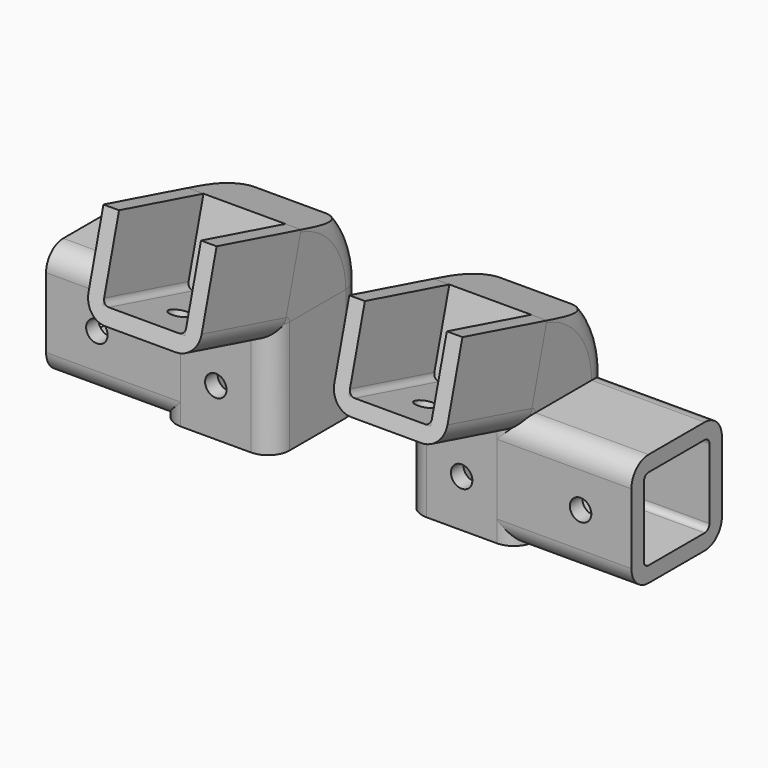
from build123d import *

# Parameters (mm, degrees)
F1_DEPTH  = 29
F3_DEPTH  = 21
F5_DEPTH  = 28
F7_DEPTH  = 28
F9_ANGLE  = 75
F11_DEPTH = 43.3
F12_R     = 2.75
F13_DEPTH = 5
F14_R     = 2.5
F15_DEPTH = 5
F16_W     = 18
F16_H     = 4
F17_DEPTH = 5.5
F18_W     = 1.5
F18_H     = 18
F19_DEPTH = 29
F21_DEPTH = 23.5
F22_R     = 2.75
F23_DEPTH = 15.2


with BuildPart() as f1:
    # F0 (on Top) → F1 (new body)
    with BuildSketch(Plane.XY):
        with BuildLine():
            Line((1.5, -4), (19.5, -4))
            ThreePointArc((19.5, -4), (23.3890872965, -2.3890872965), (25, 1.5))
            Line((25, 1.5), (25, 19.5))
            ThreePointArc((25, 19.5), (23.3890872965, 23.3890872965), (19.5, 25))
            Line((19.5, 25), (1.5, 25))
            ThreePointArc((1.5, 25), (-2.3890872965, 23.3890872965), (-4, 19.5))
            Line((-4, 19.5), (-4, 1.5))
            ThreePointArc((-4, 1.5), (-2.3890872965, -2.3890872965), (1.5, -4))
        make_face()
        with BuildLine():
            Line((19.5, 0), (1.5, 0))
            ThreePointArc((1.5, 0), (0.4393398282, 0.4393398282), (0, 1.5))
            Line((0, 1.5), (0, 19.5))
            ThreePointArc((0, 19.5), (0.4393398282, 20.5606601718), (1.5, 21))
            Line((1.5, 21), (19.5, 21))
            ThreePointArc((19.5, 21), (20.5606601718, 20.5606601718), (21, 19.5))
            Line((21, 19.5), (21, 1.5))
            ThreePointArc((21, 1.5), (20.5606601718, 0.4393398282), (19.5, 0))
        make_face(mode=Mode.SUBTRACT)
    extrude(amount=-F1_DEPTH)

    # F12 (on face) → F13 (cut)
    with BuildSketch(Plane.XZ.offset(4)):
        with Locations((10.5, -16.8672984689)):
            Circle(F12_R)
    extrude(amount=-F13_DEPTH, mode=Mode.SUBTRACT)


with BuildPart() as f3:
    # F2 (on Right) → F3 (new body)
    with BuildSketch(Plane.YZ):
        Polygon((-27.0459231361, 7.2469332629), (0, 0), (5.1763809021, 19.3185165258), (-21.869542234, 26.5654497887), align=None)
    extrude(amount=F3_DEPTH)

    # F6 (on face) → F7 (cut)
    with BuildSketch(Plane(origin=(0, -27.0459231361, 7.2469332629), x_dir=(1, 0, 0), z_dir=(0, -0.9659258263, 0.2588190451))):
        with BuildLine():
            Line((21, 20), (0, 20))
            Line((0, 20), (0, 1.5))
            ThreePointArc((0, 1.5), (0.4393398282, 0.4393398282), (1.5, 0))
            Line((1.5, 0), (19.5, 0))
            ThreePointArc((19.5, 0), (20.5606601718, 0.4393398282), (21, 1.5))
            Line((21, 1.5), (21, 20))
        make_face()
    extrude(amount=-F7_DEPTH, mode=Mode.SUBTRACT)


with BuildPart() as f5:
    # F4 (on face) → F5 (new body)
    with BuildSketch(Plane(origin=(0, -27.0459231361, 7.2469332629), x_dir=(1, 0, 0), z_dir=(0, -0.9659258263, 0.2588190451))):
        with BuildLine():
            Line((0, 1.5), (0, 20))
            Line((0, 20), (-4, 20))
            Line((-4, 20), (-4, 1.5))
            ThreePointArc((-4, 1.5), (-2.3890872965, -2.3890872965), (1.5, -4))
            Line((1.5, -4), (19.5, -4))
            ThreePointArc((19.5, -4), (23.3890872965, -2.3890872965), (25, 1.5))
            Line((25, 1.5), (25, 20))
            Line((25, 20), (21, 20))
            Line((21, 20), (21, 1.5))
            Line((21, 1.5), (21, 0))
            Line((21, 0), (19.5, 0))
            Line((19.5, 0), (1.5, 0))
            Line((1.5, 0), (0, 0))
            Line((0, 0), (0, 1.5))
        make_face()
    extrude(amount=-F5_DEPTH)

    # F14 (on face) → F15 (cut)
    with BuildSketch(Plane(origin=(0, -1.0352761804, -3.8637033052), x_dir=(1, 0, 0), z_dir=(0, -0.2588190451, -0.9659258263))):
        with Locations((10.5, 16.148366034)):
            Circle(F14_R)
    extrude(amount=-F15_DEPTH, mode=Mode.SUBTRACT)


with BuildPart() as f9:
    # F8 (on face) → F9 (revolve)
    with BuildSketch(Plane.XY):
        with BuildLine():
            ThreePointArc((0, 19.5), (0.4393398282, 20.5606601718), (1.5, 21))
            Line((1.5, 21), (19.5, 21))
            ThreePointArc((19.5, 21), (20.5606601718, 20.5606601718), (21, 19.5))
            Line((21, 19.5), (21, 1.5))
            ThreePointArc((21, 1.5), (20.5606601718, 0.4393398282), (19.5, 0))
            Line((19.5, 0), (24.7915026221, 0))
            ThreePointArc((24.7915026221, 0), (24.9476262914, 0.7427894684), (25, 1.5))
            Line((25, 1.5), (25, 19.5))
            ThreePointArc((25, 19.5), (23.3890872965, 23.3890872965), (19.5, 25))
            Line((19.5, 25), (1.5, 25))
            ThreePointArc((1.5, 25), (-2.3890872965, 23.3890872965), (-4, 19.5))
            Line((-4, 19.5), (-4, 1.5))
            ThreePointArc((-4, 1.5), (-3.9476262914, 0.7427894684), (-3.7915026221, 0))
            Line((-3.7915026221, 0), (1.5, 0))
            ThreePointArc((1.5, 0), (0.4393398282, 0.4393398282), (0, 1.5))
            Line((0, 1.5), (0, 19.5))
        make_face()
        with BuildLine():
            Line((19.5, 21), (1.5, 21))
            ThreePointArc((1.5, 21), (0.4393398282, 20.5606601718), (0, 19.5))
            Line((0, 19.5), (0, 1.5))
            ThreePointArc((0, 1.5), (0.4393398282, 0.4393398282), (1.5, 0))
            Line((1.5, 0), (19.5, 0))
            ThreePointArc((19.5, 0), (20.5606601718, 0.4393398282), (21, 1.5))
            Line((21, 1.5), (21, 19.5))
            ThreePointArc((21, 19.5), (20.5606601718, 20.5606601718), (19.5, 21))
        make_face()
    revolve(axis=Axis((10.5, 0, 0), (1, 0, 0)), revolution_arc=F9_ANGLE)

    # F10 (on face) → F11 (cut)
    with BuildSketch(Plane(origin=(-4, 0, 0), x_dir=(0, -1, 0), z_dir=(-1, 0, 0))):
        Polygon((-21.5909180111, 14.9202545633), (-5.1763809021, 19.3185165258), (-5.1763809021, 24.5526935905), (-23.506142199, 23.2962071896), align=None)
    extrude(amount=-F11_DEPTH, mode=Mode.SUBTRACT)


with BuildPart() as f17:
    # F16 (on face) → F17 (new body, symmetric)
    with BuildSketch(Plane.YZ.offset(25)):
        with Locations((10.5, -2)):
            Rectangle(F16_W, F16_H)
        with Locations((10.5, -27)):
            Rectangle(F16_W, F16_H)
        with BuildLine():
            ThreePointArc((-4, -23.5), (-2.3890872965, -27.3890872965), (1.5, -29))
            Line((1.5, -29), (1.5, -25))
            ThreePointArc((1.5, -25), (0.4393398282, -24.5606601718), (0, -23.5))
            Line((0, -23.5), (0, -5.5))
            ThreePointArc((0, -5.5), (0.4393398282, -4.4393398282), (1.5, -4))
            Line((1.5, -4), (1.5, 0))
            ThreePointArc((1.5, 0), (-2.3890872965, -1.6109127035), (-4, -5.5))
            Line((-4, -5.5), (-4, -23.5))
        make_face()
        with BuildLine():
            Line((19.5, -25), (19.5, -29))
            ThreePointArc((19.5, -29), (23.3890872965, -27.3890872965), (25, -23.5))
            Line((25, -23.5), (25, -5.5))
            ThreePointArc((25, -5.5), (23.3890872965, -1.6109127035), (19.5, 0))
            Line((19.5, 0), (19.5, -4))
            ThreePointArc((19.5, -4), (20.5606601718, -4.4393398282), (21, -5.5))
            Line((21, -5.5), (21, -23.5))
            ThreePointArc((21, -23.5), (20.5606601718, -24.5606601718), (19.5, -25))
        make_face()
    extrude(amount=F17_DEPTH, both=True)

    # F18 (on face) → F19 (cut)
    with BuildSketch(Plane(origin=(0, 0, -29), x_dir=(1, 0, 0), z_dir=(0, 0, -1))):
        with BuildLine():
            ThreePointArc((21, -1.5), (20.5606601718, -0.4393398282), (19.5, 0))
            Line((19.5, 0), (19.5, -1.5))
            Line((19.5, -1.5), (21, -1.5))
        make_face()
        with Locations((20.25, -10.5)):
            Rectangle(F18_W, F18_H)
        with BuildLine():
            Line((21, -19.5), (19.5, -19.5))
            Line((19.5, -19.5), (19.5, -21))
            ThreePointArc((19.5, -21), (20.5606601718, -20.5606601718), (21, -19.5))
        make_face()
    extrude(amount=-F19_DEPTH, mode=Mode.SUBTRACT)

    # F20 (on face) → F21 (join)
    with BuildSketch(Plane.YZ.offset(30.5)):
        with BuildLine():
            Line((25, -23.5), (25, -5.5))
            ThreePointArc((25, -5.5), (23.3890872965, -1.6109127035), (19.5, 0))
            Line((19.5, 0), (1.5, 0))
            ThreePointArc((1.5, 0), (-2.3890872965, -1.6109127035), (-4, -5.5))
            Line((-4, -5.5), (-4, -23.5))
            ThreePointArc((-4, -23.5), (-2.3890872965, -27.3890872965), (1.5, -29))
            Line((1.5, -29), (19.5, -29))
            ThreePointArc((19.5, -29), (23.3890872965, -27.3890872965), (25, -23.5))
        make_face()
        with BuildLine():
            Line((19.5, -25), (1.5, -25))
            ThreePointArc((1.5, -25), (0.4393398282, -24.5606601718), (0, -23.5))
            Line((0, -23.5), (0, -5.5))
            ThreePointArc((0, -5.5), (0.4393398282, -4.4393398282), (1.5, -4))
            Line((1.5, -4), (19.5, -4))
            ThreePointArc((19.5, -4), (20.5606601718, -4.4393398282), (21, -5.5))
            Line((21, -5.5), (21, -23.5))
            ThreePointArc((21, -23.5), (20.5606601718, -24.5606601718), (19.5, -25))
        make_face(mode=Mode.SUBTRACT)
    extrude(amount=F21_DEPTH)

    # F22 (on face) → F23 (cut)
    with BuildSketch(Plane.XZ.offset(4)):
        with Locations((40.9836284816, -14.5)):
            Circle(F22_R)
    extrude(amount=-F23_DEPTH, mode=Mode.SUBTRACT)


with BuildPart() as f25_1:
    # F25: instance of F9
    add(f9.part.mirror(Plane.YZ.offset(-21)))


with BuildPart() as f25_2:
    # F25: instance of F3
    add(f3.part.mirror(Plane.YZ.offset(-21)))


with BuildPart() as f25_3:
    # F25: instance of F17
    add(f17.part.mirror(Plane.YZ.offset(-21)))


with BuildPart() as f25_4:
    # F25: instance of F1
    add(f1.part.mirror(Plane.YZ.offset(-21)))


with BuildPart() as f25_5:
    # F25: instance of F5
    add(f5.part.mirror(Plane.YZ.offset(-21)))


solid = Compound([f1.part, f3.part, f5.part, f9.part, f17.part, f25_1.part, f25_2.part, f25_3.part, f25_4.part, f25_5.part])
